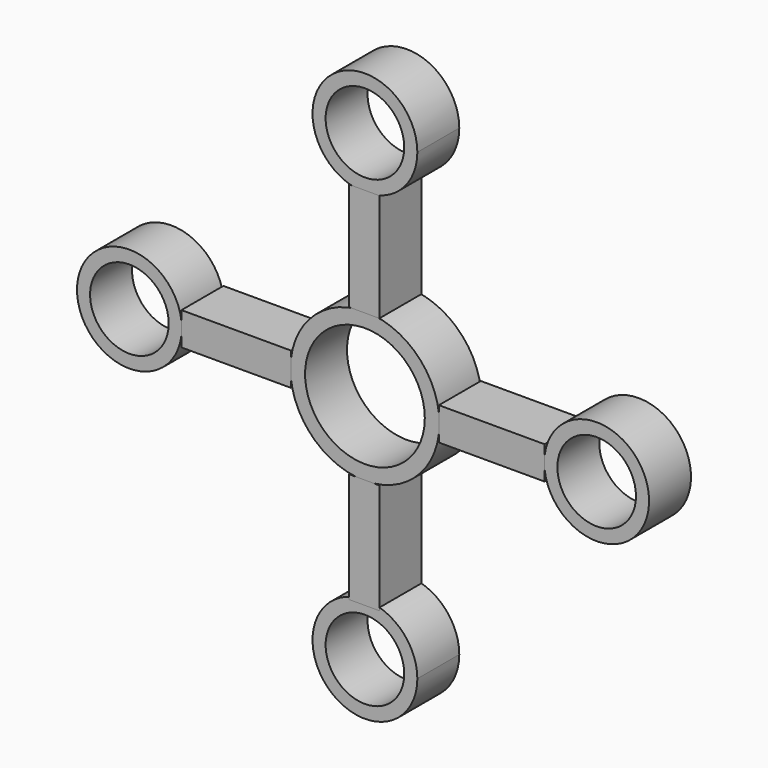
from build123d import *

# Parameters (mm, degrees)
F0_R     = 14.5061220646
F1_DEPTH = 12.7
F0_R_2   = 9.525
F0_R_3   = 12.7
F2_W     = 7.3942888994
F2_H     = 26.1644087732
F3_DEPTH = 12.7
F2_W_2   = 26.5436004847
F2_H_2   = 7.9630806576
F2_H_3   = 26.7332028598
F2_W_3   = 25.5956184119


# Not quite as in the source:
# - a feature of the source that left no trace in its solid (it failed there, or was rolled back) is left out


with BuildPart() as f1:
    # F0 (on Front) → F1 (new body)
    with BuildSketch(Plane.XZ):
        with BuildLine():
            ThreePointArc((0, -18.0544013501), (12.7663896249, -12.7663896249), (18.0544013501, 0))
            ThreePointArc((18.0544013501, 0), (12.7663896249, 12.7663896249), (0, 18.0544013501))
            ThreePointArc((0, 18.0544013501), (-12.7663896249, 12.7663896249), (-18.0544013501, 0))
            ThreePointArc((-18.0544013501, 0), (-12.7663896249, -12.7663896249), (0, -18.0544013501))
        make_face()
        Circle(F0_R, mode=Mode.SUBTRACT)
    extrude(amount=F1_DEPTH)


with BuildPart() as f1b:
    # F0 (on Front) → F1, piece 2 (new body)
    with BuildSketch(Plane.XZ):
        with BuildLine():
            ThreePointArc((12.7, -56.1544013501), (8.9802561211, -47.1741452291), (0, -43.4544013501))
            ThreePointArc((0, -43.4544013501), (-8.9802561211, -65.1346574712), (12.7, -56.1544013501))
        make_face()
        with Locations((0, -56.1544013501)):
            Circle(F0_R_2, mode=Mode.SUBTRACT)
    extrude(amount=F1_DEPTH)


with BuildPart() as f1c:
    # F0 (on Front) → F1, piece 3 (new body)
    with BuildSketch(Plane.XZ):
        with BuildLine():
            ThreePointArc((12.7, 56.1544013501), (-8.9802561211, 65.1346574712), (0, 43.4544013501))
            ThreePointArc((0, 43.4544013501), (8.9802561211, 47.1741452291), (12.7, 56.1544013501))
        make_face()
        with Locations((0, 56.1544013501)):
            Circle(F0_R_2, mode=Mode.SUBTRACT)
    extrude(amount=F1_DEPTH)


with BuildPart() as f1d:
    # F0 (on Front) → F1, piece 4 (new body)
    with BuildSketch(Plane.XZ):
        with BuildLine():
            ThreePointArc((68.8544013501, 0), (56.1544013501, 12.7), (43.4544013501, 0))
            ThreePointArc((43.4544013501, 0), (56.1544013501, -12.7), (68.8544013501, 0))
        make_face()
        with Locations((56.1544013501, 0)):
            Circle(F0_R_2, mode=Mode.SUBTRACT)
    extrude(amount=F1_DEPTH)


with BuildPart() as f1e:
    # F0 (on Front) → F1, piece 5 (new body)
    with BuildSketch(Plane.XZ):
        with Locations((-57.0763641485, 0)):
            Circle(F0_R_3)
        with Locations((-57.0763641485, 0)):
            Circle(F0_R_2, mode=Mode.SUBTRACT)
    extrude(amount=F1_DEPTH)


with BuildPart() as f3:
    # F2 (on Front) → F3 (new body)
    with BuildSketch(Plane.XZ):
        with Locations((-0.1895966707, 30.8095384389)):
            Rectangle(F2_W, F2_H)
    extrude(amount=F3_DEPTH)


with BuildPart() as f3b:
    # F2 (on Front) → F3, piece 2 (new body)
    with BuildSketch(Plane.XZ):
        with Locations((-31.1887310818, -0.09479851)):
            Rectangle(F2_W_2, F2_H_2)
    extrude(amount=F3_DEPTH)


with BuildPart() as f3c:
    # F2 (on Front) → F3, piece 3 (new body)
    with BuildSketch(Plane.XZ):
        with Locations((-0.1895966707, -31.2835322693)):
            Rectangle(F2_W, F2_H_3)
    extrude(amount=F3_DEPTH)


with BuildPart() as f3d:
    # F2 (on Front) → F3, piece 4 (new body)
    with BuildSketch(Plane.XZ):
        with Locations((30.7147400454, -0.09479851)):
            Rectangle(F2_W_3, F2_H_2)
    extrude(amount=F3_DEPTH)


solid = Compound([f1.part, f1b.part, f1c.part, f1d.part, f1e.part, f3.part, f3b.part, f3c.part, f3d.part])
